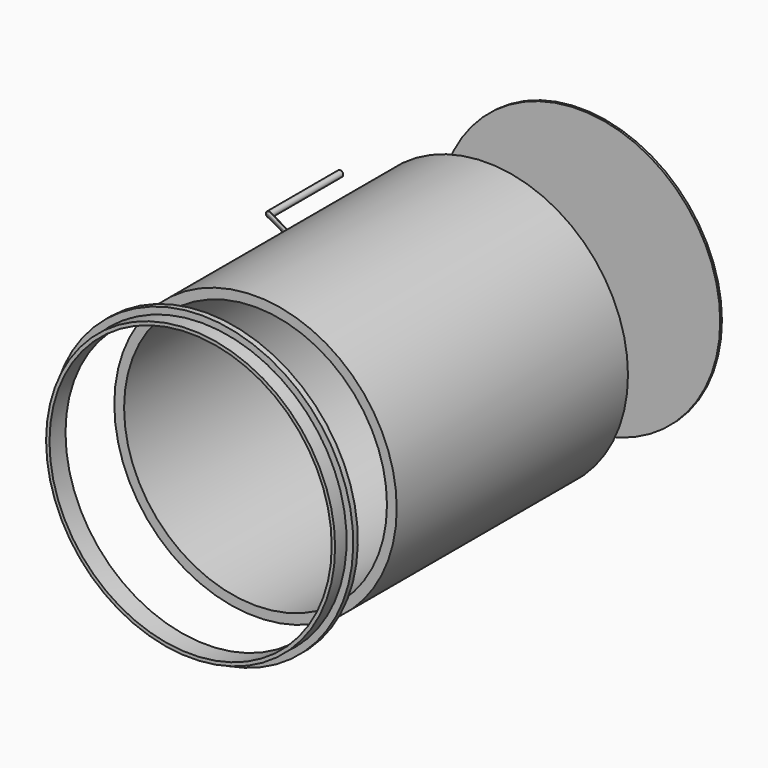
from build123d import *

# Parameters (mm, degrees)
F0_R           = 32.2649845467
F0_R_2         = 30.0329002684
F1_DEPTH       = 66.04
F3_R           = 33.02
F3_R_2         = 32.2425514632
F4_DEPTH       = 4.572
F5_W           = 1.3068169355
F5_H           = 1.5159137547
F9_R           = 32.1912372863
F10_DEPTH      = 0.4826
F11_R          = 0.6763051709
F12_DEPTH      = 33.782
F14_R          = 0.6962354259
F15_DEPTH      = 20.32
F17_DEPTH      = 0.6604
F18_DEPTH      = 0.6858
F19_T1_DEPTH   = 21.0597633564
F19_T3_DEPTH   = 21.0757959369
F19_2_T1_DEPTH = 21.0597633564
F19_2_T3_DEPTH = 21.0757959369


# Not quite as in the source:
# - a fillet or chamfer that OpenCascade refuses, or shapes differently, is made with other operations: its cross-section is extruded or revolved along the edge and cut away or added


with BuildPart() as f1:
    # F0 (on Front) → F1 (new body)
    with BuildSketch(Plane.XZ):
        Circle(F0_R)
        Circle(F0_R_2, mode=Mode.SUBTRACT)
    extrude(amount=F1_DEPTH)


with BuildPart() as f4:
    # F3 (on offset) → F4 (new body)
    with BuildSketch(Plane.XZ.offset(80.01)):
        Circle(F3_R)
        Circle(F3_R_2, mode=Mode.SUBTRACT)
    extrude(amount=F4_DEPTH)


with BuildPart() as f7:
    # F5 (on Right) → F7 (revolve)
    with BuildSketch(Plane.YZ):
        with Locations((-80.6791931391, 33.8062625378)):
            Rectangle(F5_W, F5_H)
    revolve(axis=Axis((0, -220.3602194786, 0), (0, -1, 0)))


with BuildPart() as f10:
    # F9 (on offset) → F10 (new body)
    with BuildSketch(Plane.XZ.offset(-26.924)):
        Circle(F9_R)
    extrude(amount=F10_DEPTH)


with BuildPart() as f12:
    # F11 (on Front) → F12 (new body)
    with BuildSketch(Plane.XZ):
        with Locations((-39.9328246713, 0)):
            Circle(F11_R)
    extrude(amount=F12_DEPTH)


with BuildPart() as f15:
    # F14 (on offset) → F15 (new body)
    with BuildSketch(Plane.XZ.offset(-8.382)):
        with Locations((-56.4471445978, 0)):
            Circle(F14_R)
    extrude(amount=-F15_DEPTH)


with BuildPart() as f17:
    # F16 (on Top) → F17 (new body)
    with BuildSketch(Plane.XY):
        Polygon((-39.2730757594, 0), (-55.7629354298, 8.4300749004), (-57.1569614112, 8.3933901042), (-40.630415082, 0), align=None)
    extrude(amount=F17_DEPTH)


with BuildPart() as f18:
    # F18 (new): a face of the model
    f18_faces = [f17.part.faces().sort_by_distance(p)[0] for p in [
        (-48.3112762863, 4.2598390002, 0),
    ]]
    extrude(f18_faces, amount=F18_DEPTH)

    # F19: fillet of radius 0.508 on 2 edges, made by hand

    # F19_s2 → F19_t1 (cut)
    with BuildSketch(Plane(origin=(-30.0048537502, 15.3393157701, 0), x_dir=(0, 0, 1), z_dir=(-0.8903925689, 0.455193446, 0))):
        with BuildLine():
            ThreePointArc((-0.1778, -17.876846688), (-0.5370102448, -18.0256364432), (-0.6858, -18.384846688))
            Line((-0.6858, -18.384846688), (-0.6858, -17.876846688))
            Line((-0.6858, -17.876846688), (-0.1778, -17.876846688))
        make_face()
    extrude(amount=F19_T1_DEPTH, mode=Mode.SUBTRACT)

    # F19_s4 → F19_t3 (cut)
    with BuildSketch(Plane(origin=(-49.9581715428, 25.3724168557, 0), x_dir=(0, 0, 1), z_dir=(0.8916016547, -0.4528205928, 0))):
        with BuildLine():
            ThreePointArc((-0.1778, 18.3982886432), (-0.5370102448, 18.249498888), (-0.6858, 17.8902886432))
            Line((-0.6858, 17.8902886432), (-0.6858, 18.3982886432))
            Line((-0.6858, 18.3982886432), (-0.1778, 18.3982886432))
        make_face()
    extrude(amount=F19_T3_DEPTH, mode=Mode.SUBTRACT)


with BuildPart() as f17_1:
    add(f17.part)

    # F19#2: fillet of radius 0.508 on 2 edges, made by hand

    # F19_2_s2 → F19_2_t1 (cut)
    with BuildSketch(Plane(origin=(-30.0048537502, 15.3393157701, 0), x_dir=(0, 0, 1), z_dir=(-0.8903925689, 0.455193446, 0))):
        with BuildLine():
            ThreePointArc((0.1524, -17.876846688), (0.5116102448, -18.0256364432), (0.6604, -18.384846688))
            Line((0.6604, -18.384846688), (0.6604, -17.876846688))
            Line((0.6604, -17.876846688), (0.1524, -17.876846688))
        make_face()
    extrude(amount=F19_2_T1_DEPTH, mode=Mode.SUBTRACT)

    # F19_2_s4 → F19_2_t3 (cut)
    with BuildSketch(Plane(origin=(-49.9581715428, 25.3724168557, 0), x_dir=(0, 0, 1), z_dir=(0.8916016547, -0.4528205928, 0))):
        with BuildLine():
            ThreePointArc((0.1524, 18.3982886432), (0.5116102448, 18.249498888), (0.6604, 17.8902886432))
            Line((0.6604, 17.8902886432), (0.6604, 18.3982886432))
            Line((0.6604, 18.3982886432), (0.1524, 18.3982886432))
        make_face()
    extrude(amount=F19_2_T3_DEPTH, mode=Mode.SUBTRACT)


solid = Compound([f1.part, f4.part, f7.part, f10.part, f12.part, f15.part, f18.part, f17_1.part])
